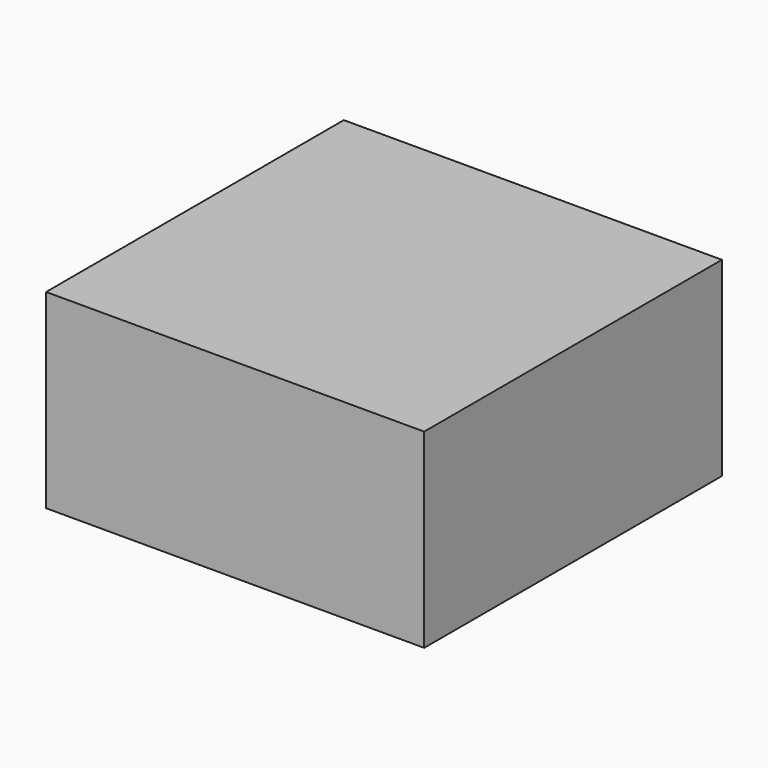
from build123d import *

# Parameters (mm, degrees)
F0_W     = 69.8630958796
F0_H     = 137.5265717506
F2_DEPTH = 70.358


# Not quite as in the source:
# - the program builds the solid bodies; features that only make, move or delete a surface that nothing else refers to are left out


with BuildPart() as f2:
    # F0 (on Top) → F2 (new body)
    with BuildSketch(Plane.XY):
        with Locations((-34.9315479398, 0)):
            Rectangle(F0_W, F0_H)
        with Locations((34.9315479398, 0)):
            Rectangle(F0_W, F0_H)
    extrude(amount=-F2_DEPTH)


solid = f2.part
